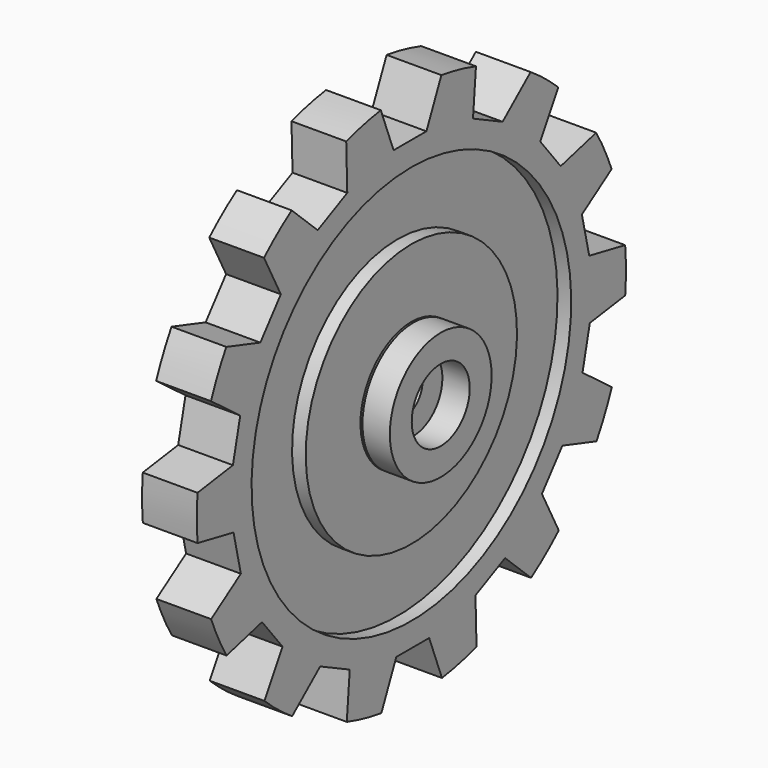
from build123d import *

# Parameters (mm, degrees)
F0_W            = 5.08
F0_H            = 5.08
F0_W_2          = 7.62
F0_H_2          = 7.62
F3_DEPTH        = 12.7
F3_COPIES_COUNT = 14


# Not quite as in the source:
# - a feature of the source that left no trace in its solid (it failed there, or was rolled back) is left out
# - a pattern or mirror of a feature is missing from the dataset's text; its kind, count and spacing are read off the source's solid


with BuildPart() as f1:
    # F0 (on Front) → F1 (revolve)
    with BuildSketch(Plane.XZ):
        with Locations((7.990129427, -21.6374768325)):
            Rectangle(F0_W, F0_H)
    revolve(axis=Axis((0.4135672934, 0, -30.9069249779), (1, 0, 0)))


with BuildPart() as f1b:
    # F0 (on Front) → F1, piece 2 (revolve)
    with BuildSketch(Plane.XZ):
        Polygon((-5.7818528368, -24.1774768325), (-5.7818528368, -19.0974768325), (-10.5137031422, -19.0974768325), (-10.8618528368, -19.0974768325), (-10.8618528368, -24.1774768325), align=None)
    revolve(axis=Axis((0.4135672934, 0, -30.9069249779), (1, 0, 0)))


with BuildPart() as f1c:
    # F0 (on Front) → F1, piece 3 (revolve)
    with BuildSketch(Plane.XZ):
        Polygon((5.08, 18.8719633837), (-5.08, 18.8719633837), (-5.08, 6.1719633837), (-2.54, 6.1719633837), (-2.54, -6.3974768325), (-5.08, -6.3974768325), (-5.08, -19.0974768325), (-3.81, -19.0974768325), (3.81, -19.0974768325), (5.08, -19.0974768325), (5.08, -6.3974768325), (2.54, -6.3974768325), (2.54, 6.1719633837), (5.08, 6.1719633837), align=None)
        with Locations((0, -22.9074768325)):
            Rectangle(F0_W_2, F0_H_2)
    revolve(axis=Axis((0.4135672934, 0, -30.9069249779), (1, 0, 0)))

    # F2 (on Right) → F3 (cut, symmetric)
    with BuildSketch(Plane.YZ):
        Polygon((-7.3202843778, 18.9508479089), (-4.1284287343, 10.6158936396), (3.4915712657, 10.6158936396), (7.2140004486, 18.9508479089), (-7.2140004486, 18.9508479089), align=None)
    f3 = extrude(amount=F3_DEPTH, both=True, mode=Mode.SUBTRACT)

    # F3_copies: F3 ×14 about axis
    f3_copies_axis = Axis((0, 0, -30.906925), (1, 0, 0))
    for i in range(1, F3_COPIES_COUNT):
        add(f3.rotate(f3_copies_axis, i * 360 / F3_COPIES_COUNT), mode=Mode.SUBTRACT)


solid = Compound([f1.part, f1b.part, f1c.part])
